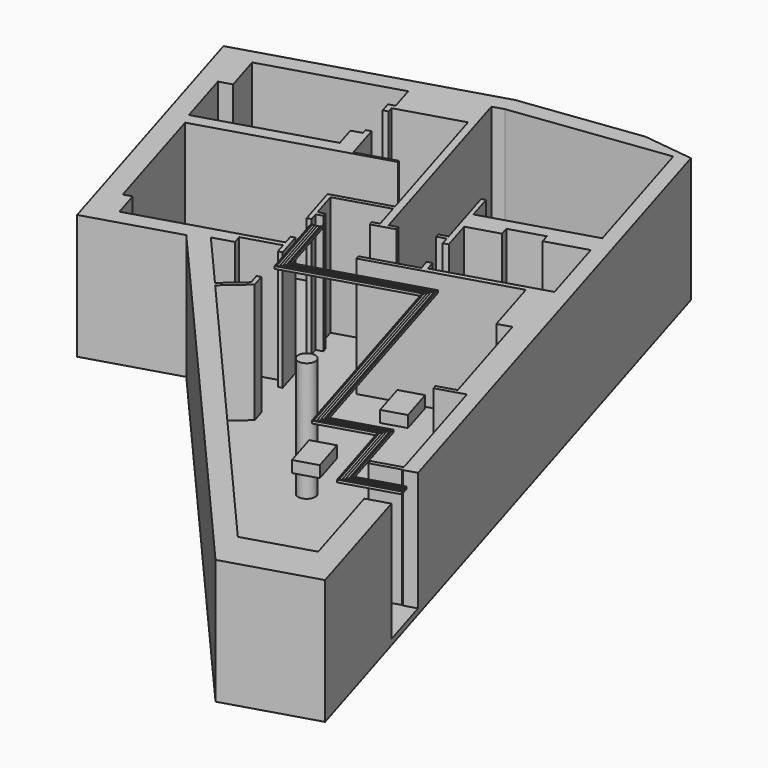
from build123d import *

# Parameters (mm, degrees)
F2_DEPTH  = 2800
F4_DEPTH  = 130
F9_DEPTH  = 270
F11_DEPTH = 270


# Not quite as in the source:
# - the dataset's text gives a spline's control points without its knots; the knots are read off the source's solid


with BuildPart() as f2:
    # F1 (on Top) → F2 (new body)
    with BuildSketch(Plane.XY):
        Polygon((8275.236689, 25028.575703), (8303.308563, 25022.239878), (8590.443808, 25109.149897), (4693.124956, 37985.198266), (3515.526115, 38130.639966), (734.613667, 37774.629948), (-4773.8228885278, 36107.3268641167), (-2682.937496, 29199.458918), (-620.098968, 29823.842444), (7849.455415, 20094.463572), (9919.6791612047, 20721.6590961385), (8971.7241505597, 23850.6338701), (8459.266294, 23695.523287), (9116.941412, 21522.845213), (7597.6430872351, 21063.0029362496), (1038.969454, 28597.264804), (1585.973667, 29073.439135), (1490.9772631837, 29387.3215373029), (1398.1364815382, 29359.2205184452), (1474.955344, 29105.400566), (975.280638, 28670.42719), (-209.293623, 30031.20426), (247.007579, 30169.347174), (187.296732, 30366.578652), (1017.231292, 30617.782986), (1093.6348589946, 30365.3352261696), (1186.4776443102, 30393.4340640164), (1003.8523771547, 30996.8554070684), (911.008887245, 30968.7562319611), (981.890957, 30734.552249), (-2157.458734, 29784.33486), (-2347.024676, 30410.491964), (-2534.665727, 30352.626467), (-3425.492361, 33295.773244), (592.95799, 34511.985947), (578.472607, 34559.843085), (-281.932544, 34299.415921), (-544.231932101, 35166.0582054976), (-658.6172266353, 35131.4381629486), (-622.797624, 35013.085332), (-861.790347, 34940.494984), (-710.00939, 34438.171176), (-3559.890774, 33575.837494), (-3973.736375, 34943.109948), (-3685.654339, 35030.306529), (-3957.948485, 35930.0042), (-1009.43758, 36822.458564), (-831.433203, 36230.915714), (-977.953063, 36186.567128), (-902.7252453764, 35938.0042036009), (-788.347823635, 35972.6218633574), (-828.961376, 36106.809831), (615.220299, 36543.934291), (1657.876463, 33099.183283), (383.018082, 32713.309544), (681.0776509064, 31728.4802572869), (773.9221048465, 31756.5796001423), (716.566381, 31946.091536), (862.5547221821, 31990.2792417169), (834.4538197544, 32083.1196385551), (688.465479, 32038.931933), (503.956941, 32648.569311), (1685.977366, 33006.342886), (1870.500849, 32396.710031), (1711.7912852511, 32348.6718696271), (1739.8921876249, 32255.8314729668), (2241.1671056465, 32407.5572092923), (2213.066203297, 32500.3976058047), (2030.3394700243, 32445.0899349197), (561.479233, 37297.943593), (817.349318, 37375.453409), (4399.014872, 37834.910601), (5411.970856, 34488.284428), (2976.110972, 33750.999116), (2796.492388, 34344.427054), (2703.651991, 34316.326151), (3165.994187, 32788.829552), (2966.7704504597, 32728.5285732888), (2994.871352927, 32635.68817651), (3194.095089, 32695.989155), (3251.4766510893, 32506.4106528712), (3366.0426838632, 32541.0840242777), (3146.687893, 33265.794326), (3864.656448, 33483.108825), (3803.840669, 33684.033369), (4569.534663, 33915.793389), (4630.341355, 33714.898868), (5539.28273, 33990.016961), (6057.785039, 32277.661675), (3664.990681, 31553.411531), (3595.992606029, 31781.3692406708), (3481.4269018349, 31746.695815678), (3556.944222, 31497.199986), (2368.648043, 31137.526868), (2396.474298, 31045.593859), (5596.857273, 32013.454034), (6018.22596, 30621.32664), (6323.550589, 30713.742204), (7106.281729, 28127.73737), (6686.088292, 28000.553351), (6714.189194, 27907.712954), (7345.901546, 28098.919452), (8246.853818, 25122.279567), (7615.1553221164, 24931.0806927414), (7643.52026, 24837.36797), align=None)
    extrude(amount=F2_DEPTH)



with BuildPart() as f2b:
    # F1 (on Top) → F2, piece 2 (new body)
    with BuildSketch(Plane.XY):
        with BuildLine():
            add(Edge.make_bspline(
                [(4051.687844, 27214.268079), (4006.094202, 27242.449275), (3955.355048, 27336.863194), (3958.583714, 27444.032762), (4014.981897, 27535.277949), (4109.397847, 27586.085124), (4216.535184, 27582.916392), (4307.722467, 27526.553999), (4358.461621, 27432.14008), (4355.232955, 27324.970513), (4298.834772, 27233.725325), (4204.418822, 27182.918151), (4097.281485, 27186.086882), (4051.687844, 27214.268079)],
                knots=[0, 0, 0, 1, 2, 3, 4, 5, 6, 7, 8, 9, 10, 11, 12, 12, 12], degree=2))
        make_face()
    extrude(amount=F2_DEPTH)


with BuildPart() as f2_1:
    add(f2.part)

    add(f2b.part)  # F4 merges F2b
    # F3 (on Top) → F4 (join)
    with BuildSketch(Plane.XY):
        Polygon((-620.098968, 29823.842444), (7849.455415, 20094.463572), (9919.6791612047, 20721.6590961385), (8971.7241505597, 23850.6338701), (8590.443808, 25109.149897), (4693.124956, 37985.198266), (3515.526115, 38130.639966), (734.613667, 37774.629948), (-4773.8228885278, 36107.3268641167), (-2682.937496, 29199.458918), align=None)
    extrude(amount=-F4_DEPTH)


with BuildPart() as f7:
    # F7: sweep along a path in F6
    with BuildLine(Plane.XY.offset(2800)) as f7_path:
        Line((8768.6126240638, 24520.5174122458), (7720.5122748463, 24203.2844155135))
        Line((7720.5122748463, 24203.2844155135), (7141.1217462707, 26117.5222835427))
        Line((7141.1217462707, 26117.5222835427), (5896.8671320517, 25740.9184399685))
        Line((5896.8671320517, 25740.9184399685), (4320.559434909, 30948.8528757533))
        Line((4320.559434909, 30948.8528757533), (1531.9500720819, 30104.7974608347))
        Line((1531.9500720819, 30104.7974608347), (1060.4484966137, 31662.5550259175))
    # F5 (on face) → F7 (sweep)
    with BuildSketch(Plane(origin=(14831.6707342136, 4489.2461027309, 0), x_dir=(-0.2897000616, 0.957117482, 0), z_dir=(0.957117482, 0.2897000616, 0))):
        with BuildLine():
            ThreePointArc((20855.8260345459, 2757.5697898865), (20830.8260345459, 2782.5697898865), (20805.8260345459, 2757.5697898865))
            ThreePointArc((20805.8260345459, 2757.5697898865), (20780.8260345459, 2782.5697898865), (20755.8260345459, 2757.5697898865))
            Line((20755.8260345459, 2757.5697898865), (20755.8260345459, 2800))
            Line((20755.8260345459, 2800), (20745.8260345459, 2800))
            Line((20745.8260345459, 2800), (20745.8260345459, 2740))
            Line((20745.8260345459, 2740), (20965.8260345459, 2740))
            Line((20965.8260345459, 2740), (20965.8260345459, 2800))
            Line((20965.8260345459, 2800), (20955.8260345459, 2800))
            Line((20955.8260345459, 2800), (20955.8260345459, 2757.5697898865))
            ThreePointArc((20955.8260345459, 2757.5697898865), (20930.8260345459, 2782.5697898865), (20905.8260345459, 2757.5697898865))
            ThreePointArc((20905.8260345459, 2757.5697898865), (20880.8260345459, 2782.5697898865), (20855.8260345459, 2757.5697898865))
        make_face()
    sweep(path=f7_path.line, transition=Transition.RIGHT)


with BuildPart() as f9:
    # F8 (on face) → F9 (new body)
    with BuildSketch(Plane.XY.offset(2800)):
        Polygon((6993.7062762883, 24222.7609520017), (6747.4612540673, 25036.310820806), (6221.0466330763, 24876.9758064276), (6467.2916552973, 24063.4259376234), align=None)
    extrude(amount=-F9_DEPTH)


with BuildPart() as f11:
    # F10 (on face) → F11 (new body)
    with BuildSketch(Plane.XY.offset(2800)):
        Polygon((7011.9703786271, 26785.8762843786), (6765.7253575562, 27599.426153531), (6239.31073634, 27440.0911398969), (6485.5557574109, 26626.5412707445), align=None)
    extrude(amount=-F11_DEPTH)


solid = Compound([f2_1.part, f7.part, f9.part, f11.part])
